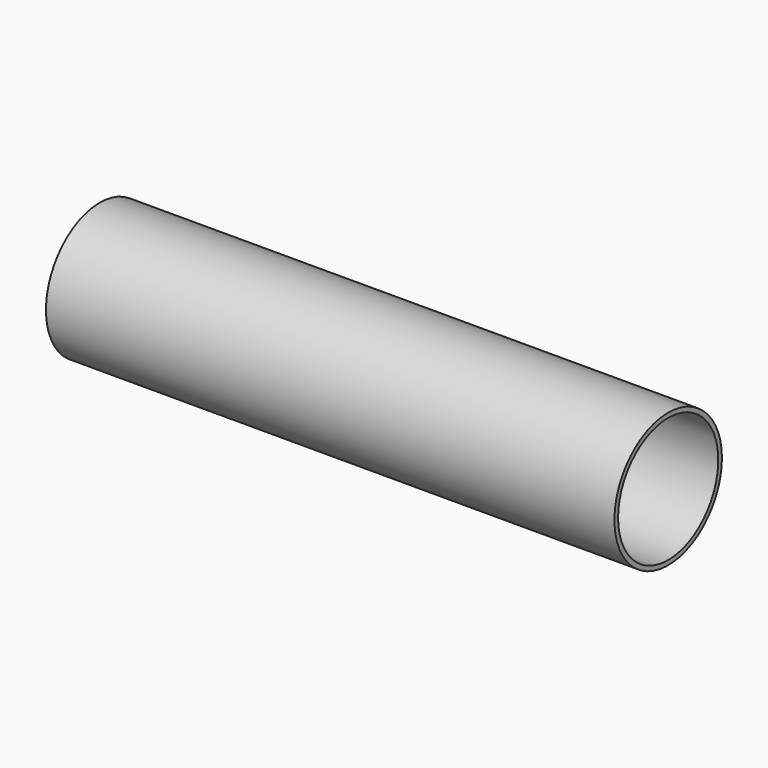
from build123d import *

# Parameters (mm, degrees)
F0_R           = 9.4567080568
F1_DEPTH       = 80
F3_D           = 17.6276
F3_CBORE_D     = 17.6276
F3_CBORE_DEPTH = 80


# Not quite as in the source:
# - the program builds the solid bodies; features that only make, move or delete a surface that nothing else refers to are left out


with BuildPart() as f1:
    # F0 (on Right) → F1 (new body)
    with BuildSketch(Plane.YZ):
        with Locations((-10.852728039, 0)):
            Circle(F0_R)
    extrude(amount=F1_DEPTH)

    # F3 (through all)
    with Locations(Plane.YZ.offset(80)):
        with Locations((-10.852728039, 0)):
            CounterBoreHole(F3_D / 2, F3_CBORE_D / 2, F3_CBORE_DEPTH)


solid = f1.part
